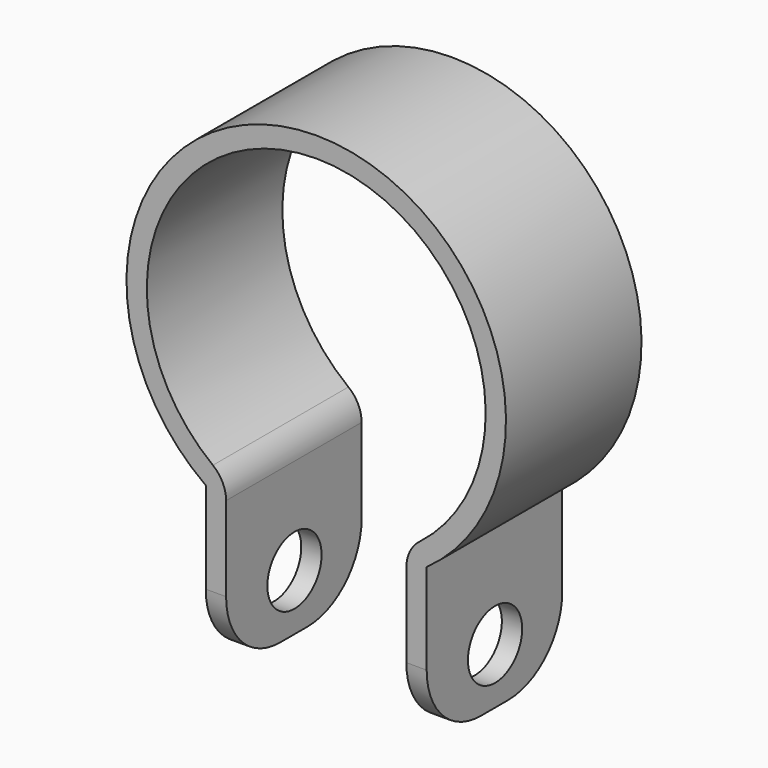
from build123d import *

# Parameters (mm, degrees)
F1_DEPTH = 25
F2_R     = 5
F3_R     = 5
F4_DEPTH = 42.9
F5_R     = 10


# Not quite as in the source:
# - a feature names something its author has since deleted; it is built from what else it names


with BuildPart() as f1:
    # F0 (on Front) → F1 (new body)
    with BuildSketch(Plane.XZ):
        with BuildLine():
            ThreePointArc((-13.2998284399, -21.1687166231), (0, 25), (13.2998284399, -21.1687166231))
            Line((13.2998284399, -21.1687166231), (13.2998284399, -46.1687166231))
            Line((13.2998284399, -46.1687166231), (16.2998284399, -46.1687166231))
            Line((16.2998284399, -46.1687166231), (16.2998284399, -22.7665454742))
            ThreePointArc((16.2998284399, -22.7665454742), (0, 28), (-16.2998284399, -22.7665454742))
            Line((-16.2998284399, -22.7665454742), (-16.2998284399, -46.2509857135))
            Line((-16.2998284399, -46.2509857135), (-13.2998284399, -46.2509857135))
            Line((-13.2998284399, -46.2509857135), (-13.2998284399, -21.1687166231))
        make_face()
    extrude(amount=F1_DEPTH)

    # F2
    f2_edges = [f1.edges().sort_by_distance(p)[0] for p in [
        (13.299828, -12.5, -21.168717),
        (-13.299828, -12.5, -21.168717),
    ]]
    fillet(f2_edges, radius=F2_R)

    # F3 (on face) → F4 (cut)
    with BuildSketch(Plane(origin=(-16.2998284399, 0, 0), x_dir=(0, -1, 0), z_dir=(-1, 0, 0))):
        with Locations((12.3893171549, -37.9563570023)):
            Circle(F3_R)
    extrude(amount=-F4_DEPTH, mode=Mode.SUBTRACT)

    # F5
    f5_edges = [f1.edges().sort_by_distance(p)[0] for p in [
        (-14.799828, 0, -46.250986),
        (-14.799828, -25, -46.250986),
        (14.799828, -25, -46.168717),
        (14.799828, 0, -46.168717),
    ]]
    fillet(f5_edges, radius=F5_R)


solid = f1.part
